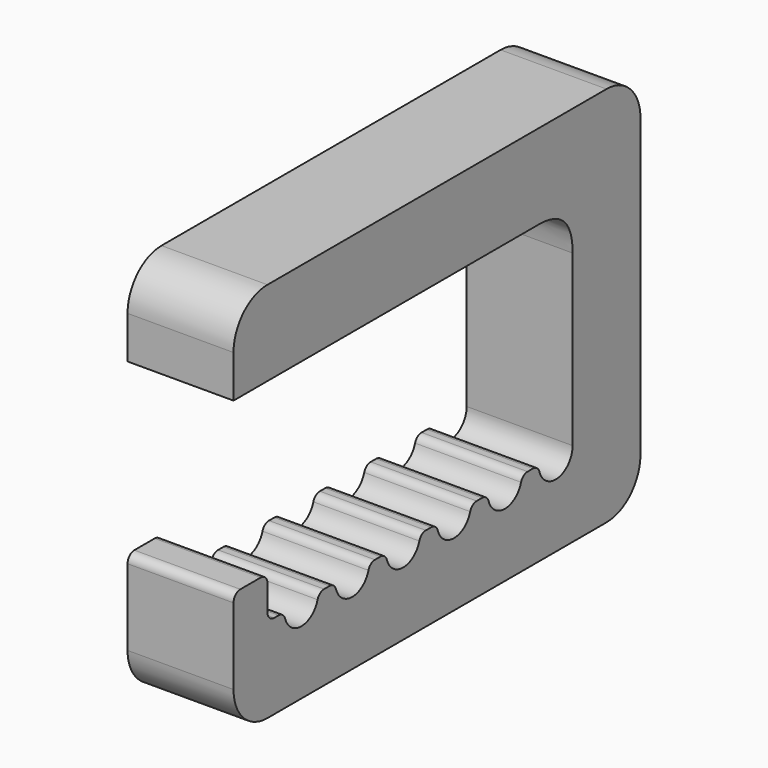
from build123d import *

# Parameters (mm, degrees)
F1_DEPTH    = 25
F2_R        = 10
F3_T1_DEPTH = 25
F4_R        = 2
F5_W        = 19
F5_H        = 10
F5_W_2      = 13
F5_H_2      = 4
F6_DEPTH    = 2


# Not quite as in the source:
# - a fillet or chamfer that OpenCascade refuses, or shapes differently, is made with other operations: its cross-section is extruded or revolved along the edge and cut away or added


with BuildPart() as f1:
    # F0 (on Right) → F1 (new body)
    with BuildSketch(Plane.YZ):
        with BuildLine():
            Line((-119.9998666872, 30.0034820876), (-120, 0))
            Line((-120, 0), (0, 0))
            Line((0, 0), (0, 90))
            Line((0, 90), (-120, 90))
            Line((-120, 90), (-120, 70))
            Line((-120, 70), (-20, 70))
            Line((-20, 70), (-20, 20.003633132))
            ThreePointArc((-20, 20.003633132), (-24.9999333448, 15.0036997872), (-29.9998666895, 20.003633132))
            Line((-29.9998666895, 20.003633132), (-34.9998666895, 20.003633132))
            ThreePointArc((-34.9998666895, 20.003633132), (-39.9998666895, 15.003633132), (-44.9998666895, 20.003633132))
            Line((-44.9998666895, 20.003633132), (-49.9998666872, 20.0034820876))
            ThreePointArc((-49.9998666872, 20.0034820876), (-54.9998666872, 15.0034820876), (-59.9998666872, 20.0034820876))
            Line((-59.9998666872, 20.0034820876), (-64.9998666872, 20.0034820876))
            ThreePointArc((-64.9998666872, 20.0034820876), (-69.9998666872, 15.0034820876), (-74.9998666872, 20.0034820876))
            Line((-74.9998666872, 20.0034820876), (-79.9998666872, 20.0034820876))
            ThreePointArc((-79.9998666872, 20.0034820876), (-84.9998666872, 15.0034820876), (-89.9998666872, 20.0034820876))
            Line((-89.9998666872, 20.0034820876), (-94.9998666872, 20.0034820876))
            ThreePointArc((-94.9998666872, 20.0034820876), (-99.9998666872, 15.0034820876), (-104.9998666872, 20.0034820876))
            Line((-104.9998666872, 20.0034820876), (-109.9998666872, 20.0034820876))
            Line((-109.9998666872, 20.0034820876), (-109.9998666872, 30.0034820876))
            Line((-109.9998666872, 30.0034820876), (-119.9998666872, 30.0034820876))
        make_face()
    extrude(amount=F1_DEPTH)

    # F2
    f2_edges = [f1.edges().sort_by_distance(p)[0] for p in [
        (12.5, -120, 90),
        (12.5, 0, 90),
        (12.5, 0, 0),
        (12.5, -120, 0),
    ]]
    fillet(f2_edges, radius=F2_R)

    # F3: fillet of radius 10 on 1 edges, made by hand

    # F3_s2 → F3_t1 (join)
    with BuildSketch(Plane.YZ):
        with BuildLine():
            add(Edge.make_bspline(
                [(-30, 70), (-20, 70), (-20, 60)],
                knots=[0, 0, 0, 1, 1, 1], degree=2, weights=[1, 1, 1]))
            Line((-20, 60), (-20, 70))
            Line((-20, 70), (-30, 70))
        make_face()
    extrude(amount=F3_T1_DEPTH)

    # F4
    f4_edges = [f1.edges().sort_by_distance(p)[0] for p in [
        (12.5, -119.999867, 30.003482),
        (12.5, -109.999867, 30.003482),
        (12.5, -109.999867, 20.003482),
        (12.5, -104.999867, 20.003482),
        (12.5, -94.999867, 20.003482),
        (12.5, -89.999867, 20.003482),
        (12.5, -79.999867, 20.003482),
        (12.5, -74.999867, 20.003482),
        (12.5, -64.999867, 20.003482),
        (12.5, -59.999867, 20.003482),
        (12.5, -49.999867, 20.003482),
        (12.5, -44.999867, 20.003633),
        (12.5, -34.999867, 20.003633),
        (12.5, -29.999867, 20.003633),
    ]]
    fillet(f4_edges, radius=F4_R)

    # F5 (on face) → F6 (join)
    with BuildSketch(Plane(origin=(0, 0, 0), x_dir=(-1, 0, 0), z_dir=(0, 1, 0))):
        Polygon((-22, 16), (-22, 13), (-3, 13), (-3, 16), (-11, 16), (-11, 21), (-3, 21), (-3, 24), (-22, 24), (-22, 21), (-14, 21), (-14, 16), align=None)
        with Locations((-12.5, 32)):
            Rectangle(F5_W, F5_H)
        with Locations((-12.5, 32)):
            Rectangle(F5_W_2, F5_H_2, mode=Mode.SUBTRACT)
        with Locations((-12.5, 45)):
            Rectangle(F5_W, F5_H)
        with Locations((-12.5, 45)):
            Rectangle(F5_W_2, F5_H_2, mode=Mode.SUBTRACT)
        Polygon((-22, 56), (-22, 53), (-3, 53), (-3, 56), (-10.7311028987, 56), (-3, 61), (-3, 64), (-12.5, 59), (-22, 64), (-22, 61), (-12.5, 56), align=None)
        Polygon((-22, 72), (-3, 65.6102970243), (-3, 68.6102970243), (-8.8134625163, 70.7304688778), (-8.5728853775, 72.4904765496), (-3, 74), (-3, 77), align=None)
    extrude(amount=F6_DEPTH)


solid = f1.part
